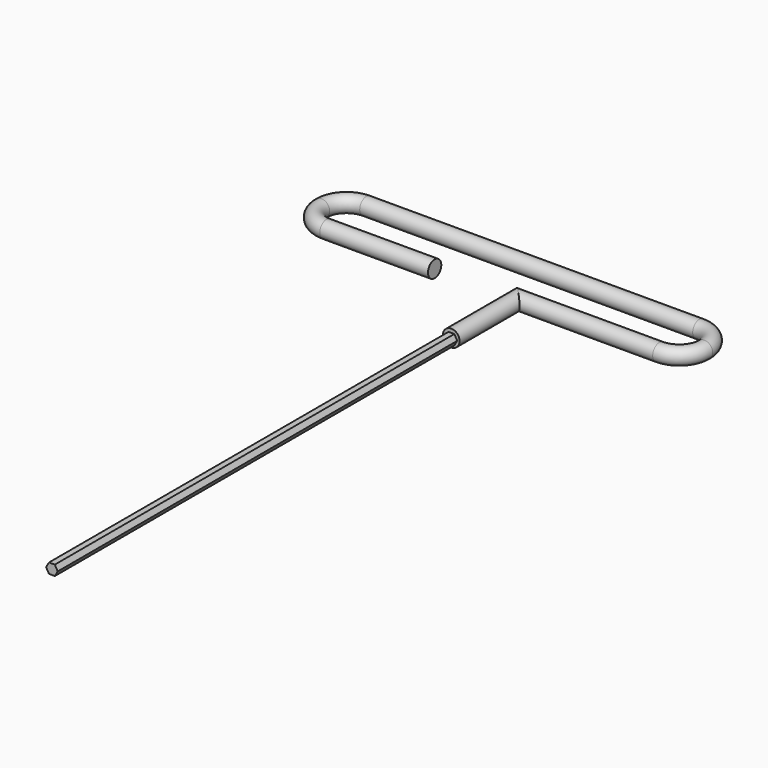
from build123d import *

# Parameters (mm, degrees)
F0_R     = 12.7
F4_DEPTH = 762


with BuildPart() as f2:
    # F2: sweep along a path in F1
    with BuildLine(Plane.XY) as f2_path:
        Line((0, 0), (0, 127))
        Line((0, 127), (215.9, 127))
        ThreePointArc((215.9, 127), (242.8407683632, 138.1592316368), (254, 165.1))
        ThreePointArc((254, 165.1), (242.8407683632, 192.0407683632), (215.9, 203.2))
        Line((215.9, 203.2), (-292.1, 203.2))
        ThreePointArc((-292.1, 203.2), (-319.0407683632, 192.0407683632), (-330.2, 165.1))
        ThreePointArc((-330.2, 165.1), (-319.0407683632, 138.1592316368), (-292.1, 127))
        Line((-292.1, 127), (-127, 127))
    # F0 (on Front) → F2 (sweep)
    with BuildSketch(Plane.XZ):
        Circle(F0_R)
    sweep(path=f2_path.line, transition=Transition.RIGHT)

    # F3 (on face) → F4 (join)
    with BuildSketch(Plane.XZ):
        Polygon((4.6947609848, 6.9345362704), (-4.1952390152, 6.9345362704), (-8.6402390152, -0.7644295692), (-4.1952390152, -8.4633954089), (4.6947609848, -8.4633954089), (9.1397609848, -0.7644295692), align=None)
    extrude(amount=F4_DEPTH)


solid = f2.part
